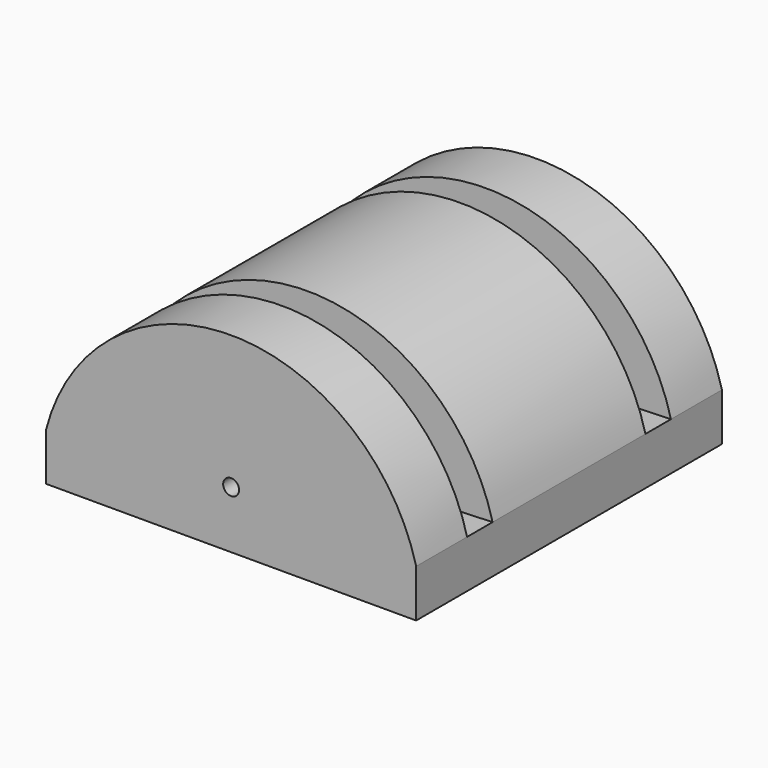
from build123d import *

# Parameters (mm, degrees)
F1_DEPTH = 76.2
F2_START = -38.1
F2_DEPTH = 12.7
F3_R     = 3.175
F4_DEPTH = 152.4


# Not quite as in the source:
# - a pattern or mirror of a feature is missing from the dataset's text; its kind, count and spacing are read off the source's solid


with BuildPart() as f1:
    # F0 (on Front) → F1 (new body, symmetric)
    with BuildSketch(Plane.XZ):
        Polygon((73.7803327453, 0), (73.7803327453, 19.05), (0, 16.51), (-73.7803327453, 19.05), (-73.7803327453, 0), align=None)
        with BuildLine():
            Line((0, 16.51), (73.7803327453, 19.05))
            ThreePointArc((73.7803327453, 19.05), (0, 76.2), (-73.7803327453, 19.05))
            Line((-73.7803327453, 19.05), (0, 16.51))
        make_face()
    extrude(amount=F1_DEPTH, both=True)

    # F0 (on Front) → F2 (cut)
    with BuildSketch(Plane.XZ.offset(F2_START)):
        with BuildLine():
            Line((0, 16.51), (73.7803327453, 19.05))
            ThreePointArc((73.7803327453, 19.05), (0, 76.2), (-73.7803327453, 19.05))
            Line((-73.7803327453, 19.05), (0, 16.51))
        make_face()
    f2 = extrude(amount=-F2_DEPTH, mode=Mode.SUBTRACT)

    # F2_copies: F2 across plane
    add(f2.mirror(Plane(origin=(0, 0, 0), x_dir=(0, 0, -1), z_dir=(0, -1, 0))), mode=Mode.SUBTRACT)

    # F3 (on face) → F4 (cut)
    with BuildSketch(Plane.XZ.offset(76.2)):
        with Locations((0, 22.86)):
            Circle(F3_R)
    extrude(amount=-F4_DEPTH, mode=Mode.SUBTRACT)


solid = f1.part
